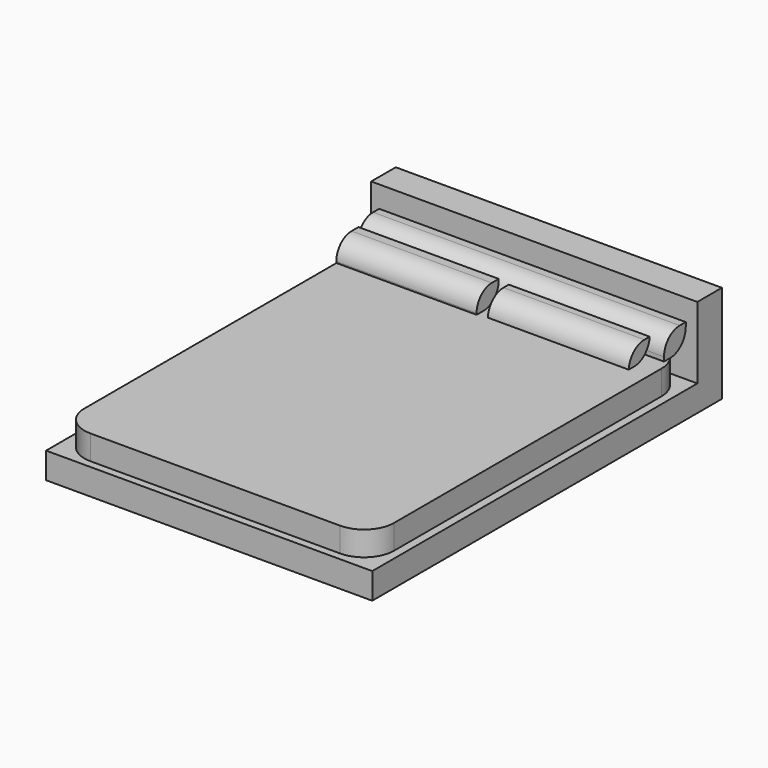
from build123d import *

# Parameters (mm, degrees)
F0_W         = 1524
F0_H         = 2042.16
F1_DEPTH     = 121.92
F2_W         = 1446.9777941704
F2_H         = 1841.9745564461
F3_DEPTH     = 114.3
F4_R         = 139.8119358242
F5_W         = 1524
F5_H         = 143.4489317703
F6_DEPTH     = 335.28
F7_W         = 126.9334554672
F7_H         = 111.0667288303
F8_DEPTH     = 716.28
F9_R         = 91.44
F10_W        = 122.4000453949
F10_H        = 86.1333906651
F11_DEPTH    = 658.368
F12_T1_DEPTH = 1114.797444092
F14_W        = 129.2001008987
F14_H        = 95.2000617981
F15_DEPTH    = 655.32
F16_R        = 88.392


# Not quite as in the source:
# - a fillet or chamfer that OpenCascade refuses, or shapes differently, is made with other operations: its cross-section is extruded or revolved along the edge and cut away or added


with BuildPart() as f1:
    # F0 (on Top) → F1 (new body)
    with BuildSketch(Plane.XY):
        Rectangle(F0_W, F0_H)
    extrude(amount=F1_DEPTH)

    # F2 (on face) → F3 (join)
    with BuildSketch(Plane.XY.offset(121.92)):
        with Locations((-2.98023e-05, -64.4892752171)):
            Rectangle(F2_W, F2_H)
    extrude(amount=F3_DEPTH)

    # F4
    f4_edges = [f1.edges().sort_by_distance(p)[0] for p in [
        (-723.488927, 856.498003, 179.07),
        (723.488867, 856.498003, 179.07),
        (723.488867, -985.476553, 179.07),
        (-723.488927, -985.476553, 179.07),
    ]]
    fillet(f4_edges, radius=F4_R)

    # F5 (on face) → F6 (join)
    with BuildSketch(Plane.XY.offset(121.92)):
        with Locations((0, 949.3555341148)):
            Rectangle(F5_W, F5_H)
    extrude(amount=F6_DEPTH)


with BuildPart() as f8:
    # F7 (on Right) → F8 (new body, symmetric)
    with BuildSketch(Plane.YZ):
        with Locations((803.5338521004, 308.3667308092)):
            Rectangle(F7_W, F7_H)
    extrude(amount=F8_DEPTH, both=True)

    # F9
    f9_edges = [f8.edges().sort_by_distance(p)[0] for p in [
        (0, 740.067124, 363.900095),
        (0, 867.00058, 252.833366),
    ]]
    fillet(f9_edges, radius=F9_R)


with BuildPart() as f11:
    # F10 (on Right) → F11 (new body)
    with BuildSketch(Plane.YZ):
        with Locations((667.5337553024, 298.1667369604)):
            Rectangle(F10_W, F10_H)
    extrude(amount=F11_DEPTH)

    # F12: fillet of radius 91.44 on 2 edges, made by hand

    # F12_s2 → F12_t1 (cut)
    with BuildSketch(Plane.YZ.offset(-228.214722046)):
        with BuildLine():
            ThreePointArc((697.6196214234, 341.2334322929), (634.8659870967, 316.3009880952), (606.333732605, 255.1000416279))
            Line((606.333732605, 255.1000416279), (606.333732605, 341.2334322929))
            Line((606.333732605, 341.2334322929), (697.6196214234, 341.2334322929))
        make_face()
        with BuildLine():
            ThreePointArc((728.7337779999, 341.2334322929), (700.2015235081, 280.0324858256), (637.4478891815, 255.1000416279))
            Line((637.4478891815, 255.1000416279), (728.7337779999, 255.1000416279))
            Line((728.7337779999, 255.1000416279), (728.7337779999, 341.2334322929))
        make_face()
    extrude(amount=F12_T1_DEPTH, mode=Mode.SUBTRACT)


with BuildPart() as f15:
    # F14 (on offset) → F15 (new body)
    with BuildSketch(Plane.YZ.offset(-704.088)):
        with Locations((666.4004325867, 300.3335297108)):
            Rectangle(F14_W, F14_H)
    extrude(amount=F15_DEPTH)

    # F16
    f16_edges = [f15.edges().sort_by_distance(p)[0] for p in [
        (-376.428, 601.800382, 347.933561),
        (-376.428, 731.000483, 252.733499),
    ]]
    fillet(f16_edges, radius=F16_R)


solid = Compound([f1.part, f8.part, f11.part, f15.part])
